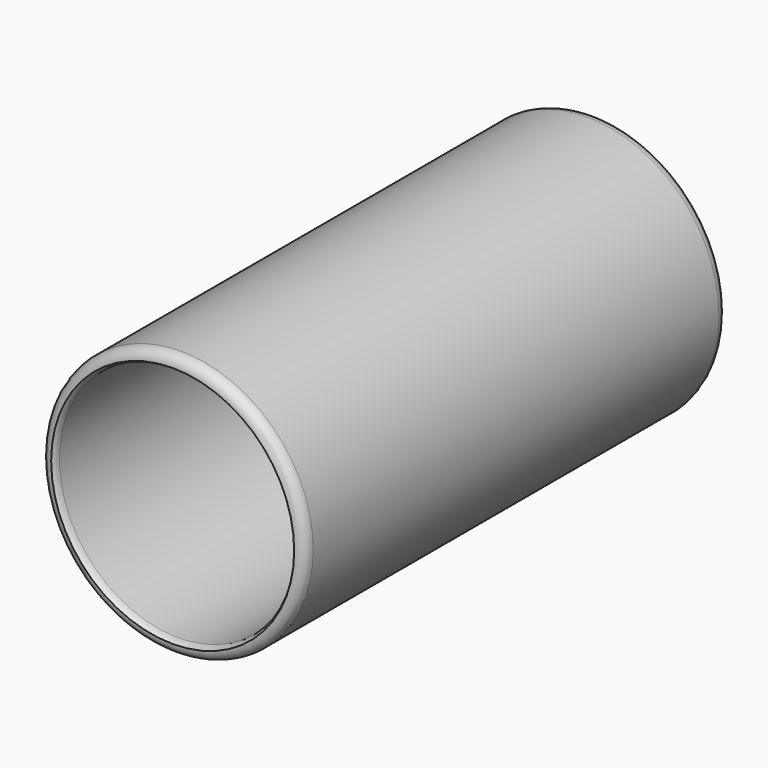
from build123d import *

# Parameters (mm, degrees)
F0_R     = 25
F1_DEPTH = 100
F2_T     = -2.5
F3_R     = 2


# Not quite as in the source:
# - a fillet or chamfer that OpenCascade refuses, or shapes differently, is made with other operations: its cross-section is extruded or revolved along the edge and cut away or added


with BuildPart() as f1:
    # F0 (on Front) → F1 (new body)
    with BuildSketch(Plane.XZ):
        Circle(F0_R)
    extrude(amount=F1_DEPTH)

    # F2
    f2_openings = [f1.faces().sort_by_distance(p)[0] for p in [
        (0, -100, 0),
    ]]
    offset(amount=F2_T, openings=f2_openings)

    # F3
    f3_edges = [f1.edges().sort_by_distance(p)[0] for p in [
        (25, -50, 0),
        (-25, 0, 0),
        (-25, -100, 0),
    ]]
    fillet(f3_edges, radius=F3_R)

    # F4: fillet of radius 2 on 3 edges, made by hand

    # F4_s1 → F4_t2 (revolve)
    with BuildSketch(Plane.XY):
        with BuildLine():
            ThreePointArc((22.5, -4.5), (21.9142135624, -3.0857864376), (20.5, -2.5))
            Line((20.5, -2.5), (22.5, -2.5))
            Line((22.5, -2.5), (22.5, -4.5))
        make_face()
    revolve(axis=Axis((0, -2.5, 0), (0, 1, 0)))

    # F4_s3 → F4_t4 (revolve, cut)
    with BuildSketch(Plane.XY):
        with BuildLine():
            ThreePointArc((23, -100), (22.6291713066, -99.3842311257), (22.5, -98.6771243445))
            Line((22.5, -98.6771243445), (22.5, -100))
            Line((22.5, -100), (23, -100))
        make_face()
    revolve(axis=Axis((0, -100, 0), (0, -1, 0)), mode=Mode.SUBTRACT)


solid = f1.part
